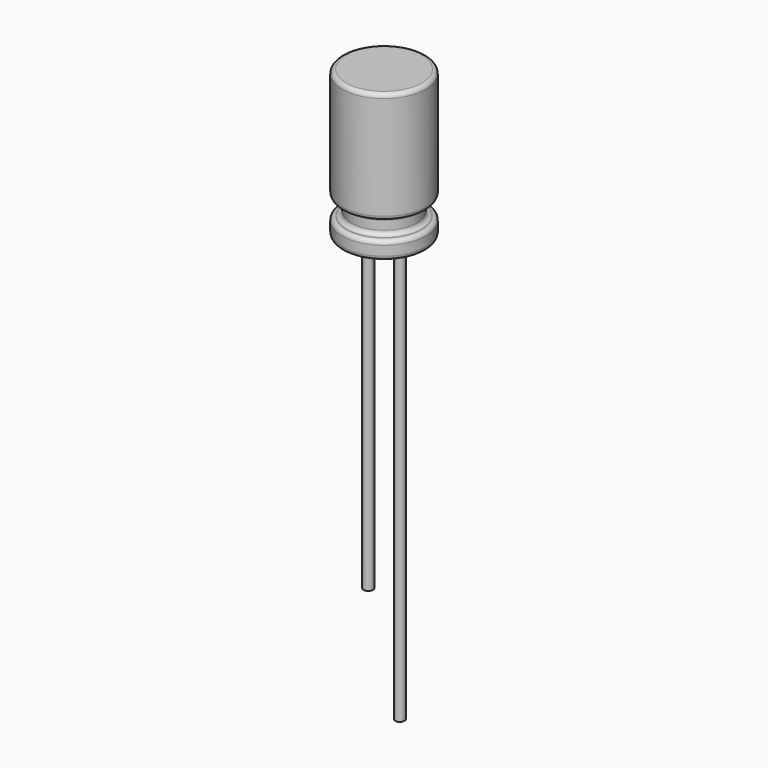
from build123d import *

# Parameters (mm, degrees)
F0_R     = 2
F1_DEPTH = 7
F2_W     = 1.194575103
F2_H     = 0.820221263
F4_R     = 0.2
F5_R     = 0.225
F6_DEPTH = 15
F7_DEPTH = 20


with BuildPart() as f1:
    # F0 (on Top) → F1 (new body)
    with BuildSketch(Plane.XY):
        Circle(F0_R)
    extrude(amount=F1_DEPTH)

    # F2 (on Front) → F3 (revolve, cut)
    with BuildSketch(Plane.XZ):
        with Locations((2.1560959285, 1.2628298136)):
            Rectangle(F2_W, F2_H)
    revolve(axis=Axis((0, 0, 0), (0, 0, -1)), mode=Mode.SUBTRACT)

    # F4
    f4_edges = [f1.edges().sort_by_distance(p)[0] for p in [
        (-2, 0, 7),
        (-2, 0, 1.67294),
        (-1.558808, 0, 1.67294),
        (-2, 0, 0.852719),
        (-2, 0, 0),
        (-1.558808, 0, 0.852719),
    ]]
    fillet(f4_edges, radius=F4_R)

    # F5 (on face) → F6 (join)
    with BuildSketch(Plane(origin=(0, 0, 0), x_dir=(1, 0, 0), z_dir=(0, 0, -1))):
        with Locations((-0.75, 0)):
            Circle(F5_R)
    extrude(amount=F6_DEPTH)

    # F5 (on face) → F7 (join)
    with BuildSketch(Plane(origin=(0, 0, 0), x_dir=(1, 0, 0), z_dir=(0, 0, -1))):
        with BuildLine():
            ThreePointArc((0.975, 0), (0.75, 0.225), (0.525, 0))
            ThreePointArc((0.525, 0), (0.75, -0.225), (0.975, 0))
        make_face()
    extrude(amount=F7_DEPTH)


solid = f1.part
